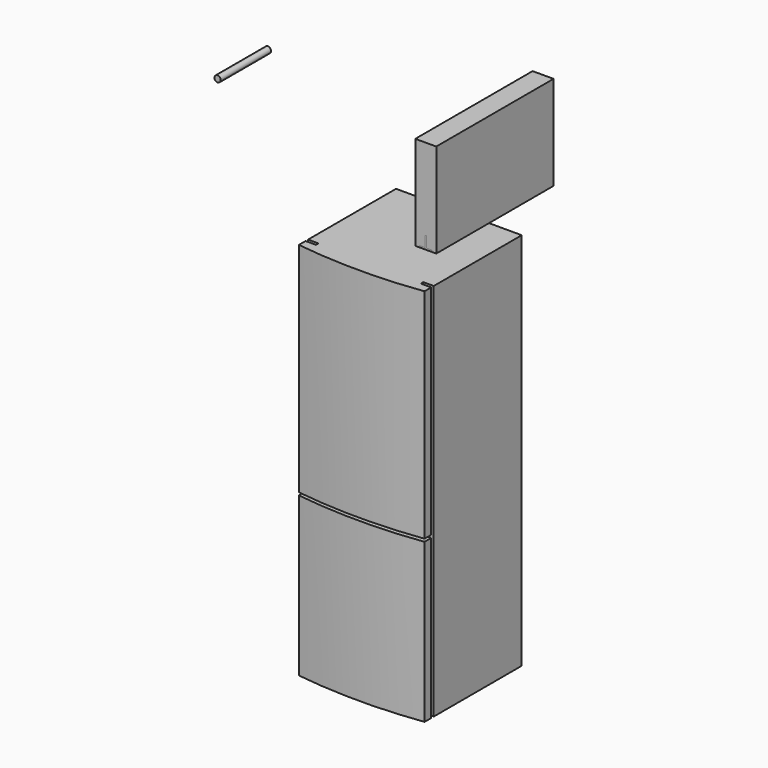
from build123d import *

# Parameters (mm, degrees)
F5_DEPTH  = 700
F6_DEPTH  = 700
F7_R      = 15
F8_DEPTH  = 300
F12_DEPTH = 1810
F13_W     = 75
F13_H     = 13
F14_DEPTH = 600


# Not quite as in the source:
# - the program builds the solid bodies; features that only make, move or delete a surface that nothing else refers to are left out


with BuildPart() as f5:
    # F4 (on Front) → F5 (new body)
    with BuildSketch(Plane.XZ):
        Polygon((100, 2540), (0, 2540), (0, 2090), (20, 2090), (20, 2098), (46, 2098), (46, 2150), (54, 2150), (54, 2098), (80, 2098), (80, 2090), (100, 2090), align=None)
    extrude(amount=F5_DEPTH)


with BuildPart() as f6:
    # F4 (on Front) → F6 (new body, through all)
    with BuildSketch(Plane.XZ):
        Polygon((20, 2098), (20, 2090), (80, 2090), (80, 2098), (54, 2098), (54, 2150), (46, 2150), (46, 2098), align=None)
    extrude(amount=F6_DEPTH)


with BuildPart() as f8:
    # F7 (on Front) → F8 (new body)
    with BuildSketch(Plane.XZ):
        with Locations((-932, 2495)):
            Circle(F7_R)
    extrude(amount=F8_DEPTH)


with BuildPart() as f8_1:
    # F9: moved
    add(f8.part.moved(Location((0, -415, 0))))


with BuildPart() as f12:
    # F11 (on offset) → F12 (new body)
    with BuildSketch(Plane.XY.offset(50)):
        with BuildLine():
            Line((-20, -565), (-20, -40))
            Line((-20, -40), (-620, -40))
            Line((-620, -40), (-620, -565))
            Line((-620, -565), (-570, -565))
            Line((-570, -565), (-570, -580))
            Line((-570, -580), (-620, -580))
            Line((-620, -580), (-620, -620))
            ThreePointArc((-620, -620), (-320, -640), (-20, -620))
            Line((-20, -620), (-20, -580))
            Line((-20, -580), (-70, -580))
            Line((-70, -580), (-70, -565))
            Line((-70, -565), (-20, -565))
        make_face()
    extrude(amount=F12_DEPTH)

    # F13 (on face) → F14 (cut, through all)
    with BuildSketch(Plane.YZ.offset(-20)):
        with Locations((-602.5, 813.5)):
            Rectangle(F13_W, F13_H)
    extrude(amount=-F14_DEPTH, mode=Mode.SUBTRACT)


solid = Compound([f5.part, f6.part, f8_1.part, f12.part])
